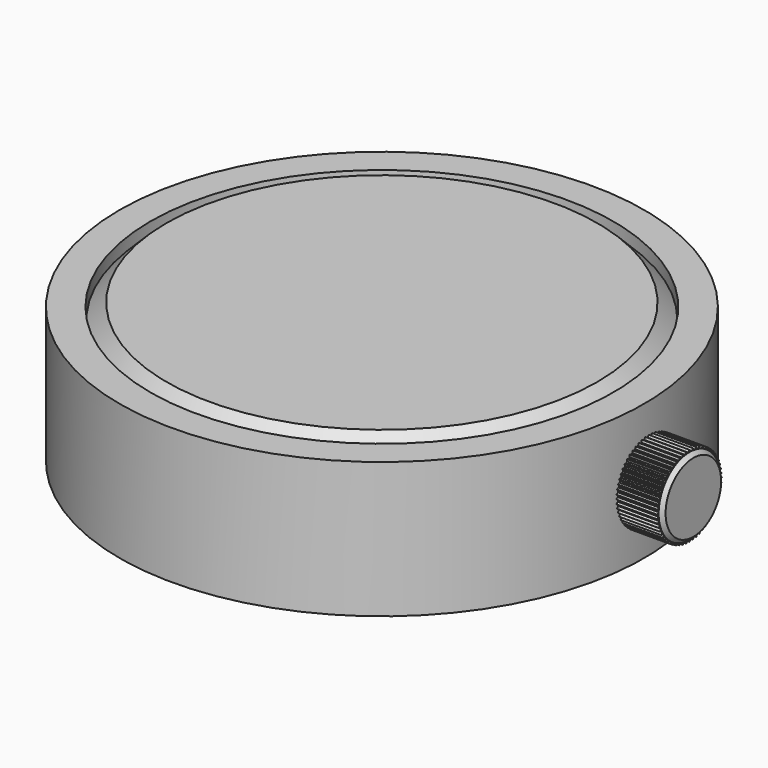
from build123d import *

# Parameters (mm, degrees)
F0_R      = 16
F1_DEPTH  = 5.7
F2_R      = 14.95
F3_DEPTH  = 1.35
F4_R      = 14.95
F5_DEPTH  = 0.7
F7_R      = 1.44
F8_DEPTH  = 1.78
F9_R      = 2.5
F10_DEPTH = 2.9
F11_SIZE  = 0.25
F12_SIZE  = 1
F15_DEPTH = 2.65
F16_COUNT = 60


# Not quite as in the source:
# - a fillet or chamfer that OpenCascade refuses, or shapes differently, is made with other operations: its cross-section is extruded or revolved along the edge and cut away or added


with BuildPart() as f1:
    # F0 (on Top) → F1 (new body)
    with BuildSketch(Plane.XY):
        Circle(F0_R)
    extrude(amount=F1_DEPTH)

    # F2 (on face) → F3 (join)
    with BuildSketch(Plane.XY.offset(5.7)):
        Circle(F2_R)
    extrude(amount=F3_DEPTH)

    # F4 (on face) → F5 (join)
    with BuildSketch(Plane(origin=(0, 0, 0), x_dir=(1, 0, 0), z_dir=(0, 0, -1))):
        Circle(F4_R)
    extrude(amount=F5_DEPTH)

    # F12
    f12_edges = [f1.edges().sort_by_distance(p)[0] for p in [
        (-14.95, 0, 7.05),
    ]]
    chamfer(f12_edges, length=F12_SIZE)

    # F13: fillet of radius 1 on 1 edges, made by hand

    # F13_s1 → F13_t2 (revolve, cut)
    with BuildSketch(Plane.XZ):
        with BuildLine():
            ThreePointArc((14.95, 0), (14.5876687769, -0.5062257748), (13.9960607986, -0.7))
            Line((13.9960607986, -0.7), (14.95, -0.7))
            Line((14.95, -0.7), (14.95, 0))
        make_face()
    revolve(axis=Axis((0, 0, -0.7), (0, 0, -1)), mode=Mode.SUBTRACT)


with BuildPart() as f8:
    # F7 (on offset) → F8 (new body)
    with BuildSketch(Plane.YZ.offset(15.5)):
        with Locations((0, 2.5)):
            Circle(F7_R)
    extrude(amount=F8_DEPTH)


with BuildPart() as f10:
    # F9 (on face) → F10 (new body)
    with BuildSketch(Plane.YZ.offset(17.28)):
        with Locations((0, 2.5)):
            Circle(F9_R)
    extrude(amount=F10_DEPTH)

    # F11
    f11_edges = [f10.edges().sort_by_distance(p)[0] for p in [
        (20.18, -2.5, 2.5),
    ]]
    chamfer(f11_edges, length=F11_SIZE)


with BuildPart() as f15:
    # F14 (on face) → F15 (new body)
    with BuildSketch(Plane(origin=(17.28, 0, 0), x_dir=(0, -1, 0), z_dir=(-1, 0, 0))):
        Polygon((-2.473188857, 2.405332807), (-2.473187466, 2.5947035277), (-2.6249994986, 2.4983775031), align=None)
    extrude(amount=-F15_DEPTH)


with BuildPart() as f16_1:
    # F16: instance of F15
    add(f15.part.rotate(Axis((17.28, 0, 2.5), (-1, 0, 0)), 1 * 360 / F16_COUNT))


with BuildPart() as f16_2:
    # F16: instance of F15
    add(f15.part.rotate(Axis((17.28, 0, 2.5), (-1, 0, 0)), 2 * 360 / F16_COUNT))


with BuildPart() as f16_3:
    # F16: instance of F15
    add(f15.part.rotate(Axis((17.28, 0, 2.5), (-1, 0, 0)), 3 * 360 / F16_COUNT))


with BuildPart() as f16_4:
    # F16: instance of F15
    add(f15.part.rotate(Axis((17.28, 0, 2.5), (-1, 0, 0)), 4 * 360 / F16_COUNT))


with BuildPart() as f16_5:
    # F16: instance of F15
    add(f15.part.rotate(Axis((17.28, 0, 2.5), (-1, 0, 0)), 5 * 360 / F16_COUNT))


with BuildPart() as f16_6:
    # F16: instance of F15
    add(f15.part.rotate(Axis((17.28, 0, 2.5), (-1, 0, 0)), 6 * 360 / F16_COUNT))


with BuildPart() as f16_7:
    # F16: instance of F15
    add(f15.part.rotate(Axis((17.28, 0, 2.5), (-1, 0, 0)), 7 * 360 / F16_COUNT))


with BuildPart() as f16_8:
    # F16: instance of F15
    add(f15.part.rotate(Axis((17.28, 0, 2.5), (-1, 0, 0)), 8 * 360 / F16_COUNT))


with BuildPart() as f16_9:
    # F16: instance of F15
    add(f15.part.rotate(Axis((17.28, 0, 2.5), (-1, 0, 0)), 9 * 360 / F16_COUNT))


with BuildPart() as f16_10:
    # F16: instance of F15
    add(f15.part.rotate(Axis((17.28, 0, 2.5), (-1, 0, 0)), 10 * 360 / F16_COUNT))


with BuildPart() as f16_11:
    # F16: instance of F15
    add(f15.part.rotate(Axis((17.28, 0, 2.5), (-1, 0, 0)), 11 * 360 / F16_COUNT))


with BuildPart() as f16_12:
    # F16: instance of F15
    add(f15.part.rotate(Axis((17.28, 0, 2.5), (-1, 0, 0)), 12 * 360 / F16_COUNT))


with BuildPart() as f16_13:
    # F16: instance of F15
    add(f15.part.rotate(Axis((17.28, 0, 2.5), (-1, 0, 0)), 13 * 360 / F16_COUNT))


with BuildPart() as f16_14:
    # F16: instance of F15
    add(f15.part.rotate(Axis((17.28, 0, 2.5), (-1, 0, 0)), 14 * 360 / F16_COUNT))


with BuildPart() as f16_15:
    # F16: instance of F15
    add(f15.part.rotate(Axis((17.28, 0, 2.5), (-1, 0, 0)), 15 * 360 / F16_COUNT))


with BuildPart() as f16_16:
    # F16: instance of F15
    add(f15.part.rotate(Axis((17.28, 0, 2.5), (-1, 0, 0)), 16 * 360 / F16_COUNT))


with BuildPart() as f16_17:
    # F16: instance of F15
    add(f15.part.rotate(Axis((17.28, 0, 2.5), (-1, 0, 0)), 17 * 360 / F16_COUNT))


with BuildPart() as f16_18:
    # F16: instance of F15
    add(f15.part.rotate(Axis((17.28, 0, 2.5), (-1, 0, 0)), 18 * 360 / F16_COUNT))


with BuildPart() as f16_19:
    # F16: instance of F15
    add(f15.part.rotate(Axis((17.28, 0, 2.5), (-1, 0, 0)), 19 * 360 / F16_COUNT))


with BuildPart() as f16_20:
    # F16: instance of F15
    add(f15.part.rotate(Axis((17.28, 0, 2.5), (-1, 0, 0)), 20 * 360 / F16_COUNT))


with BuildPart() as f16_21:
    # F16: instance of F15
    add(f15.part.rotate(Axis((17.28, 0, 2.5), (-1, 0, 0)), 21 * 360 / F16_COUNT))


with BuildPart() as f16_22:
    # F16: instance of F15
    add(f15.part.rotate(Axis((17.28, 0, 2.5), (-1, 0, 0)), 22 * 360 / F16_COUNT))


with BuildPart() as f16_23:
    # F16: instance of F15
    add(f15.part.rotate(Axis((17.28, 0, 2.5), (-1, 0, 0)), 23 * 360 / F16_COUNT))


with BuildPart() as f16_24:
    # F16: instance of F15
    add(f15.part.rotate(Axis((17.28, 0, 2.5), (-1, 0, 0)), 24 * 360 / F16_COUNT))


with BuildPart() as f16_25:
    # F16: instance of F15
    add(f15.part.rotate(Axis((17.28, 0, 2.5), (-1, 0, 0)), 25 * 360 / F16_COUNT))


with BuildPart() as f16_26:
    # F16: instance of F15
    add(f15.part.rotate(Axis((17.28, 0, 2.5), (-1, 0, 0)), 26 * 360 / F16_COUNT))


with BuildPart() as f16_27:
    # F16: instance of F15
    add(f15.part.rotate(Axis((17.28, 0, 2.5), (-1, 0, 0)), 27 * 360 / F16_COUNT))


with BuildPart() as f16_28:
    # F16: instance of F15
    add(f15.part.rotate(Axis((17.28, 0, 2.5), (-1, 0, 0)), 28 * 360 / F16_COUNT))


with BuildPart() as f16_29:
    # F16: instance of F15
    add(f15.part.rotate(Axis((17.28, 0, 2.5), (-1, 0, 0)), 29 * 360 / F16_COUNT))


with BuildPart() as f16_30:
    # F16: instance of F15
    add(f15.part.rotate(Axis((17.28, 0, 2.5), (-1, 0, 0)), 30 * 360 / F16_COUNT))


with BuildPart() as f16_31:
    # F16: instance of F15
    add(f15.part.rotate(Axis((17.28, 0, 2.5), (-1, 0, 0)), 31 * 360 / F16_COUNT))


with BuildPart() as f16_32:
    # F16: instance of F15
    add(f15.part.rotate(Axis((17.28, 0, 2.5), (-1, 0, 0)), 32 * 360 / F16_COUNT))


with BuildPart() as f16_33:
    # F16: instance of F15
    add(f15.part.rotate(Axis((17.28, 0, 2.5), (-1, 0, 0)), 33 * 360 / F16_COUNT))


with BuildPart() as f16_34:
    # F16: instance of F15
    add(f15.part.rotate(Axis((17.28, 0, 2.5), (-1, 0, 0)), 34 * 360 / F16_COUNT))


with BuildPart() as f16_35:
    # F16: instance of F15
    add(f15.part.rotate(Axis((17.28, 0, 2.5), (-1, 0, 0)), 35 * 360 / F16_COUNT))


with BuildPart() as f16_36:
    # F16: instance of F15
    add(f15.part.rotate(Axis((17.28, 0, 2.5), (-1, 0, 0)), 36 * 360 / F16_COUNT))


with BuildPart() as f16_37:
    # F16: instance of F15
    add(f15.part.rotate(Axis((17.28, 0, 2.5), (-1, 0, 0)), 37 * 360 / F16_COUNT))


with BuildPart() as f16_38:
    # F16: instance of F15
    add(f15.part.rotate(Axis((17.28, 0, 2.5), (-1, 0, 0)), 38 * 360 / F16_COUNT))


with BuildPart() as f16_39:
    # F16: instance of F15
    add(f15.part.rotate(Axis((17.28, 0, 2.5), (-1, 0, 0)), 39 * 360 / F16_COUNT))


with BuildPart() as f16_40:
    # F16: instance of F15
    add(f15.part.rotate(Axis((17.28, 0, 2.5), (-1, 0, 0)), 40 * 360 / F16_COUNT))


with BuildPart() as f16_41:
    # F16: instance of F15
    add(f15.part.rotate(Axis((17.28, 0, 2.5), (-1, 0, 0)), 41 * 360 / F16_COUNT))


with BuildPart() as f16_42:
    # F16: instance of F15
    add(f15.part.rotate(Axis((17.28, 0, 2.5), (-1, 0, 0)), 42 * 360 / F16_COUNT))


with BuildPart() as f16_43:
    # F16: instance of F15
    add(f15.part.rotate(Axis((17.28, 0, 2.5), (-1, 0, 0)), 43 * 360 / F16_COUNT))


with BuildPart() as f16_44:
    # F16: instance of F15
    add(f15.part.rotate(Axis((17.28, 0, 2.5), (-1, 0, 0)), 44 * 360 / F16_COUNT))


with BuildPart() as f16_45:
    # F16: instance of F15
    add(f15.part.rotate(Axis((17.28, 0, 2.5), (-1, 0, 0)), 45 * 360 / F16_COUNT))


with BuildPart() as f16_46:
    # F16: instance of F15
    add(f15.part.rotate(Axis((17.28, 0, 2.5), (-1, 0, 0)), 46 * 360 / F16_COUNT))


with BuildPart() as f16_47:
    # F16: instance of F15
    add(f15.part.rotate(Axis((17.28, 0, 2.5), (-1, 0, 0)), 47 * 360 / F16_COUNT))


with BuildPart() as f16_48:
    # F16: instance of F15
    add(f15.part.rotate(Axis((17.28, 0, 2.5), (-1, 0, 0)), 48 * 360 / F16_COUNT))


with BuildPart() as f16_49:
    # F16: instance of F15
    add(f15.part.rotate(Axis((17.28, 0, 2.5), (-1, 0, 0)), 49 * 360 / F16_COUNT))


with BuildPart() as f16_50:
    # F16: instance of F15
    add(f15.part.rotate(Axis((17.28, 0, 2.5), (-1, 0, 0)), 50 * 360 / F16_COUNT))


with BuildPart() as f16_51:
    # F16: instance of F15
    add(f15.part.rotate(Axis((17.28, 0, 2.5), (-1, 0, 0)), 51 * 360 / F16_COUNT))


with BuildPart() as f16_52:
    # F16: instance of F15
    add(f15.part.rotate(Axis((17.28, 0, 2.5), (-1, 0, 0)), 52 * 360 / F16_COUNT))


with BuildPart() as f16_53:
    # F16: instance of F15
    add(f15.part.rotate(Axis((17.28, 0, 2.5), (-1, 0, 0)), 53 * 360 / F16_COUNT))


with BuildPart() as f16_54:
    # F16: instance of F15
    add(f15.part.rotate(Axis((17.28, 0, 2.5), (-1, 0, 0)), 54 * 360 / F16_COUNT))


with BuildPart() as f16_55:
    # F16: instance of F15
    add(f15.part.rotate(Axis((17.28, 0, 2.5), (-1, 0, 0)), 55 * 360 / F16_COUNT))


with BuildPart() as f16_56:
    # F16: instance of F15
    add(f15.part.rotate(Axis((17.28, 0, 2.5), (-1, 0, 0)), 56 * 360 / F16_COUNT))


with BuildPart() as f16_57:
    # F16: instance of F15
    add(f15.part.rotate(Axis((17.28, 0, 2.5), (-1, 0, 0)), 57 * 360 / F16_COUNT))


with BuildPart() as f16_58:
    # F16: instance of F15
    add(f15.part.rotate(Axis((17.28, 0, 2.5), (-1, 0, 0)), 58 * 360 / F16_COUNT))


with BuildPart() as f16_59:
    # F16: instance of F15
    add(f15.part.rotate(Axis((17.28, 0, 2.5), (-1, 0, 0)), 59 * 360 / F16_COUNT))


with BuildPart() as f18:
    # F17 (on Front) → F18 (revolve)
    with BuildSketch(Plane.XZ):
        with BuildLine():
            Line((-16.1, 5.8), (-15, 5.8))
            Line((-15, 5.8), (-15, 6.8))
            Line((-15, 6.8), (-17, 6.8))
            Line((-17, 6.8), (-17, -2))
            Line((-17, -2), (0, -2))
            Line((0, -2), (0, -0.8))
            Line((0, -0.8), (-13.9960607986, -0.8))
            ThreePointArc((-13.9960607986, -0.8), (-14.6165444809, -0.6082951062), (-15.0207558752, -0.1))
            Line((-15.0207558752, -0.1), (-16.1, -0.1))
            Line((-16.1, -0.1), (-16.1, 5.8))
        make_face()
    revolve(axis=Axis((0, 0, -1.4), (0, 0, -1)))


solid = Compound([f1.part, f8.part, f10.part, f15.part, f16_1.part, f16_2.part, f16_3.part, f16_4.part, f16_5.part, f16_6.part, f16_7.part, f16_8.part, f16_9.part, f16_10.part, f16_11.part, f16_12.part, f16_13.part, f16_14.part, f16_15.part, f16_16.part, f16_17.part, f16_18.part, f16_19.part, f16_20.part, f16_21.part, f16_22.part, f16_23.part, f16_24.part, f16_25.part, f16_26.part, f16_27.part, f16_28.part, f16_29.part, f16_30.part, f16_31.part, f16_32.part, f16_33.part, f16_34.part, f16_35.part, f16_36.part, f16_37.part, f16_38.part, f16_39.part, f16_40.part, f16_41.part, f16_42.part, f16_43.part, f16_44.part, f16_45.part, f16_46.part, f16_47.part, f16_48.part, f16_49.part, f16_50.part, f16_51.part, f16_52.part, f16_53.part, f16_54.part, f16_55.part, f16_56.part, f16_57.part, f16_58.part, f16_59.part, f18.part])
